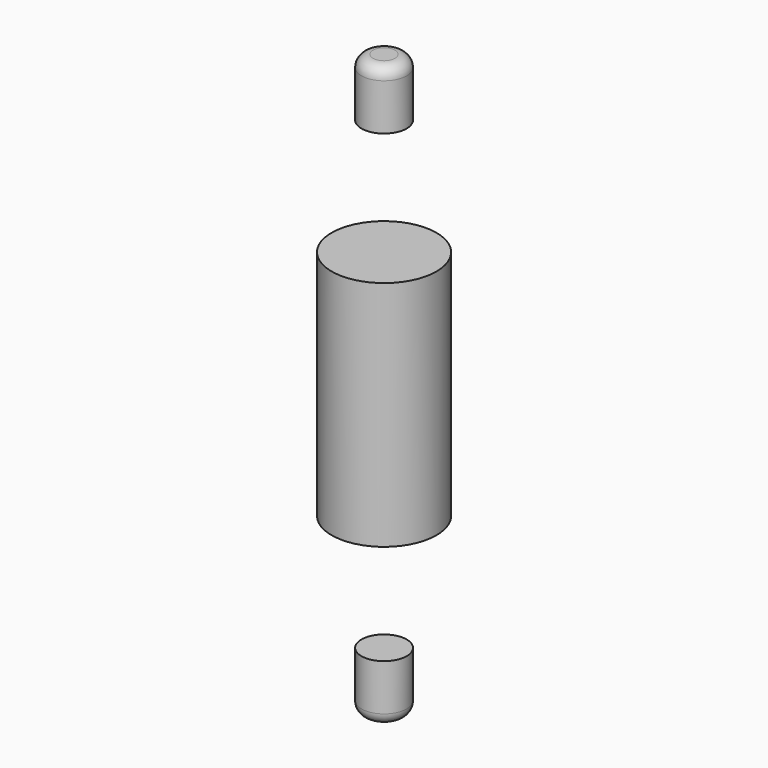
from build123d import *

# Parameters (mm, degrees)
F0_R     = 22.5696692522
F1_DEPTH = 100
F7_R     = 9.7379485752
F8_DEPTH = 25
F9_R     = 5


# Not quite as in the source:
# - a feature of the source that left no trace in its solid (it failed there, or was rolled back) is left out
# - the program builds the solid bodies; features that only make, move or delete a surface that nothing else refers to are left out


with BuildPart() as f1:
    # F0 (on Top) → F1 (new body)
    with BuildSketch(Plane.XY):
        Circle(F0_R)
    extrude(amount=F1_DEPTH)


with BuildPart() as f8:
    # F7 (on offset) → F8 (new body)
    with BuildSketch(Plane.XY.offset(150)):
        Circle(F7_R)
    extrude(amount=F8_DEPTH)

    # F9
    f9_edges = [f8.edges().sort_by_distance(p)[0] for p in [
        (-9.737949, 0, 175),
    ]]
    fillet(f9_edges, radius=F9_R)


with BuildPart() as f10_1:
    # F10: instance of F8
    add(f8.part.mirror(Plane.XY.offset(50)))


solid = Compound([f1.part, f8.part, f10_1.part])
